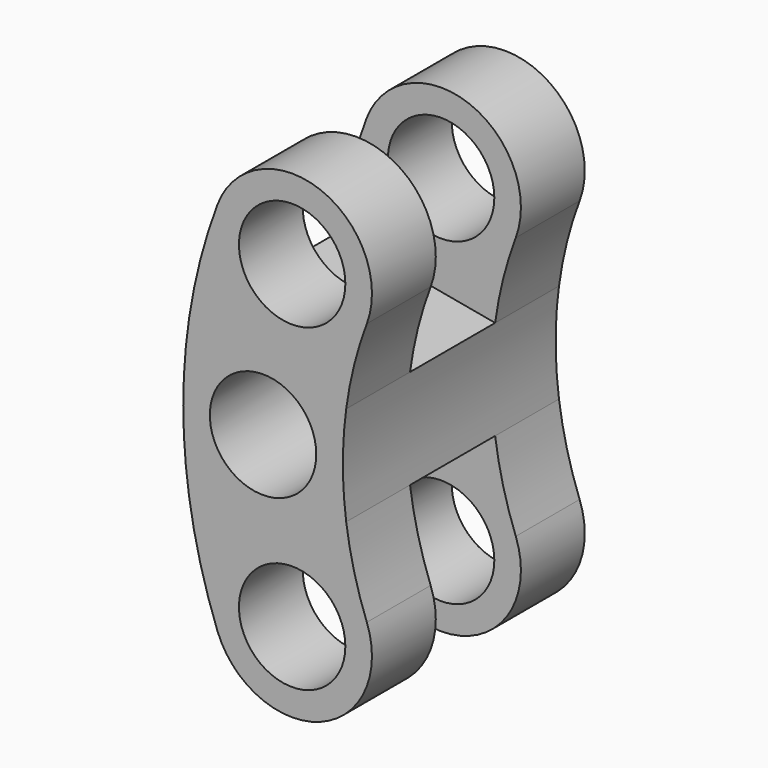
from build123d import *

# Parameters (mm, degrees)
F0_R     = 5
F1_DEPTH = 12.5
F2_DEPTH = 5


# Not quite as in the source:
# - a feature of the source that left no trace in its solid (it failed there, or was rolled back) is left out


with BuildPart() as f1:
    # F0 (on Front) → F1 (new body, symmetric)
    with BuildSketch(Plane.XZ):
        with BuildLine():
            ThreePointArc((5.0784583206, 4.6742255002), (5.8300100803, 8.5686007088), (7.0173413473, 12.3529411765))
            ThreePointArc((7.0173413473, 12.3529411765), (2.6470588235, 22.0173413473), (-7.0173413473, 17.6470588235))
            ThreePointArc((-7.0173413473, 17.6470588235), (-8.6271086588, 12.5781627487), (-9.6893672694, 7.3669570477))
            Line((-9.6893672694, 7.3669570477), (5.0784583206, 4.6742255002))
        make_face()
        with Locations((0, 15)):
            Circle(F0_R, mode=Mode.SUBTRACT)
        with BuildLine():
            ThreePointArc((5.0784583206, -4.6742255002), (4.7649343015, 0), (5.0784583206, 4.6742255002))
            Line((5.0784583206, 4.6742255002), (-9.6893672694, 7.3669570477))
            ThreePointArc((-9.6893672694, 7.3669570477), (-10.2350656985, 0), (-9.6893672694, -7.3669570477))
            Line((-9.6893672694, -7.3669570477), (5.0784583206, -4.6742255002))
        make_face()
        with Locations((-2.7350656985, 0)):
            Circle(F0_R, mode=Mode.SUBTRACT)
        with BuildLine():
            ThreePointArc((7.0173413473, -12.3529411765), (5.8300100803, -8.5686007088), (5.0784583206, -4.6742255002))
            Line((5.0784583206, -4.6742255002), (-9.6893672694, -7.3669570477))
            ThreePointArc((-9.6893672694, -7.3669570477), (-8.6271086588, -12.5781627487), (-7.0173413473, -17.6470588235))
            ThreePointArc((-7.0173413473, -17.6470588235), (2.6470588235, -22.0173413473), (7.0173413473, -12.3529411765))
        make_face()
        with Locations((0, -15)):
            Circle(F0_R, mode=Mode.SUBTRACT)
    extrude(amount=F1_DEPTH, both=True)

    # F0 (on Front) → F2 (cut, symmetric)
    with BuildSketch(Plane.XZ):
        with BuildLine():
            ThreePointArc((5.0784583206, 4.6742255002), (5.8300100803, 8.5686007088), (7.0173413473, 12.3529411765))
            ThreePointArc((7.0173413473, 12.3529411765), (2.6470588235, 22.0173413473), (-7.0173413473, 17.6470588235))
            ThreePointArc((-7.0173413473, 17.6470588235), (-8.6271086588, 12.5781627487), (-9.6893672694, 7.3669570477))
            Line((-9.6893672694, 7.3669570477), (5.0784583206, 4.6742255002))
        make_face()
        with Locations((0, 15)):
            Circle(F0_R, mode=Mode.SUBTRACT)
        with BuildLine():
            ThreePointArc((7.0173413473, -12.3529411765), (5.8300100803, -8.5686007088), (5.0784583206, -4.6742255002))
            Line((5.0784583206, -4.6742255002), (-9.6893672694, -7.3669570477))
            ThreePointArc((-9.6893672694, -7.3669570477), (-8.6271086588, -12.5781627487), (-7.0173413473, -17.6470588235))
            ThreePointArc((-7.0173413473, -17.6470588235), (2.6470588235, -22.0173413473), (7.0173413473, -12.3529411765))
        make_face()
        with Locations((0, -15)):
            Circle(F0_R, mode=Mode.SUBTRACT)
    extrude(amount=F2_DEPTH, both=True, mode=Mode.SUBTRACT)


solid = f1.part
